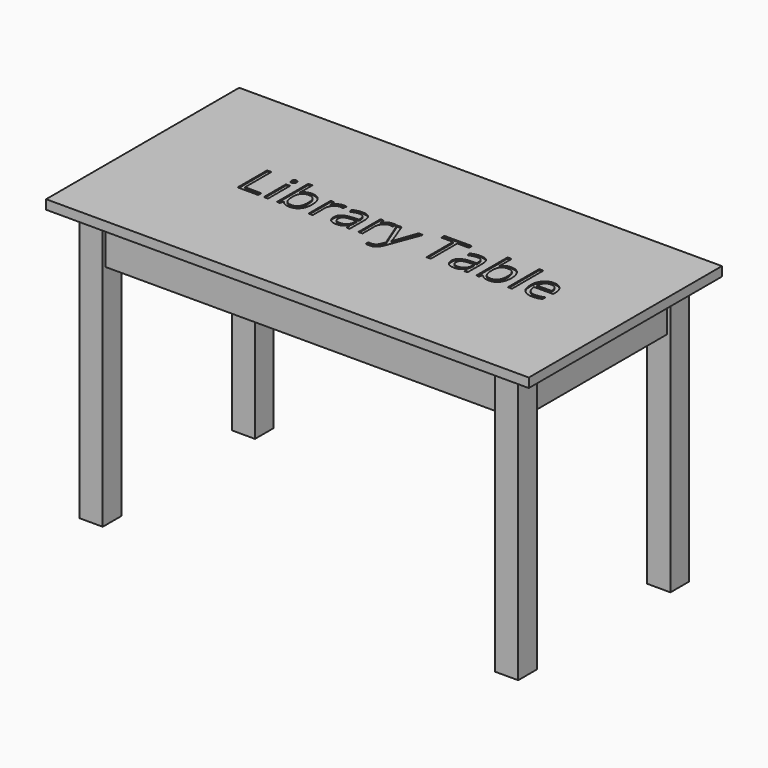
from build123d import *

# Parameters (mm, degrees)
F0_W          = 63.5
F0_H          = 63.5
F1_DEPTH      = 736.6
F2_W          = 1320.8
F2_H          = 660.4
F3_DEPTH      = 25.4
F4_W          = 19.6524569765
F4_H          = 114.7871199608
F5_DEPTH      = 1076.96
F8_W          = 19.4317102432
F8_H          = 115.1752654076
F9_DEPTH      = 1079.5
F10_W         = 17.9119110107
F10_H         = 117.9186883926
F11_DEPTH     = 477.52
F12_TEXT_SIZE = 141.3007991181
F13_DEPTH     = 3.175


# Not quite as in the source:
# - a feature of the source that left no trace in its solid (it failed there, or was rolled back) is left out
# - a length typed as a fraction of an inch, garbled in the dataset ("3 / 203.2 mm" for 3/8 in), is restored
# - Text() gives the source's letters only with a copy of the font that has no kerning and outlines rounded to 1/6400 em; it was checked with that copy


with BuildPart() as f1:
    # F0 (on Top) → F1 (new body)
    with BuildSketch(Plane.XY):
        with Locations((31.75, 31.75)):
            Rectangle(F0_W, F0_H)
    extrude(amount=F1_DEPTH)


with BuildPart() as f1b:
    # F0 (on Top) → F1, piece 2 (new body)
    with BuildSketch(Plane.XY):
        with Locations((1168.4, 31.75)):
            Rectangle(F0_W, F0_H)
    extrude(amount=F1_DEPTH)


with BuildPart() as f1c:
    # F0 (on Top) → F1, piece 3 (new body)
    with BuildSketch(Plane.XY):
        with Locations((31.75, 552.45)):
            Rectangle(F0_W, F0_H)
    extrude(amount=F1_DEPTH)


with BuildPart() as f1d:
    # F0 (on Top) → F1, piece 4 (new body)
    with BuildSketch(Plane.XY):
        with Locations((1168.4, 552.45)):
            Rectangle(F0_W, F0_H)
    extrude(amount=F1_DEPTH)


with BuildPart() as f3:
    # F2 (on face) → F3 (new body)
    with BuildSketch(Plane.XY.offset(736.6)):
        with Locations((596.9, 295.148)):
            Rectangle(F2_W, F2_H)
    extrude(amount=F3_DEPTH)

    # F12 (on face) → F13 (cut)
    with BuildSketch(Plane.XY.offset(762)):
        with Locations((208.0593407154, 263.2475197315)):
            Text('Library Table', F12_TEXT_SIZE, font='Open Sans', text_align=(TextAlign.LEFT, TextAlign.BOTTOM))
    extrude(amount=-F13_DEPTH, mode=Mode.SUBTRACT)


with BuildPart() as f5:
    # F4 (on face) → F5 (new body)
    with BuildSketch(Plane.YZ.offset(63.5)):
        with Locations((19.4888352416, 679.2064400196)):
            Rectangle(F4_W, F4_H)
    extrude(amount=F5_DEPTH)


with BuildPart() as f9:
    # F8 (on face) → F9 (new body)
    with BuildSketch(Plane(origin=(1136.65, 0, 0), x_dir=(0, -1, 0), z_dir=(-1, 0, 0))):
        with Locations((-564.5701885223, 679.0123672962)):
            Rectangle(F8_W, F8_H)
    extrude(amount=F9_DEPTH)


with BuildPart() as f11:
    # F10 (on face) → F11 (new body)
    with BuildSketch(Plane(origin=(0, 63.5, 0), x_dir=(-1, 0, 0), z_dir=(0, 1, 0))):
        with Locations((-1182.2068691254, 677.6406558037)):
            Rectangle(F10_W, F10_H)
    extrude(amount=F11_DEPTH)


solid = Compound([f1.part, f1b.part, f1c.part, f1d.part, f3.part, f5.part, f9.part, f11.part])
